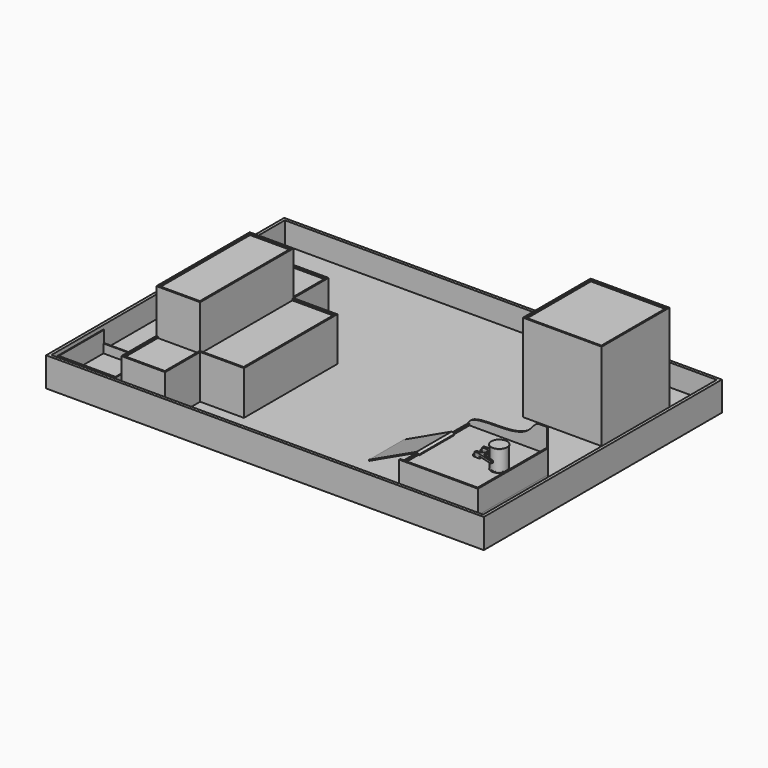
from build123d import *

# Parameters (mm, degrees)
F0_R      = 27.2
F1_DEPTH  = 2.83
F2_R      = 26.4
F3_DEPTH  = 67.36
F4_R      = 27.2
F5_DEPTH  = 2.83
F9_W      = 270
F9_H      = 300
F10_DEPTH = 72
F12_DEPTH = 15
F14_DEPTH = 5
F15_W     = 5
F15_H     = 290
F16_DEPTH = 5
F17_W     = 1500
F17_H     = 1020
F18_DEPTH = 25
F19_W     = 270
F19_H     = 290
F20_DEPTH = 300
F21_W     = 260
F21_H     = 280
F22_DEPTH = 5
F23_W     = 1500
F23_H     = 1020
F23_W_2   = 1480
F23_H_2   = 1000
F24_DEPTH = 75
F26_DEPTH = 150
F27_W     = 150
F27_H     = 400
F28_DEPTH = 150
F29_W     = 140
F29_H     = 390
F30_DEPTH = 5
F31_W     = 140
F31_H     = 145
F31_W_2   = 145
F31_H_2   = 390
F32_DEPTH = 5
F33_R     = 3
F34_DEPTH = 4
F35_R     = 3.99999
F35_2_R   = 3.99999
F36_R     = 3
F37_DEPTH = 8
F38_R     = 3
F39_DEPTH = 8
F40_R     = 3
F40_R_2   = 2.5
F41_DEPTH = 3
F42_R     = 3
F42_R_2   = 2.5
F43_DEPTH = 3
F45_DEPTH = 270.001
F46_W     = 200
F46_H     = 200
F46_W_2   = 194
F46_H_2   = 191
F47_DEPTH = 30
F49_DEPTH = 40
F52_DEPTH = 75
F50_R     = 2.5
F50_R_2   = 2.5911728926
F53_DEPTH = 7.25
F46_W_3   = 270
F46_H_3   = 300


# Not quite as in the source:
# - a fillet or chamfer is up to 0.001 mm smaller than in the source, because OpenCascade refuses the exact size
# - a feature names something its author has since deleted; it is built from what else it names


with BuildPart() as f1:
    # F0 (on Top) → F1 (new body)
    with BuildSketch(Plane.XY):
        Circle(F0_R)
    extrude(amount=F1_DEPTH)

    # F2 (on face) → F3 (join)
    with BuildSketch(Plane.XY.offset(2.83)):
        Circle(F2_R)
    extrude(amount=F3_DEPTH)

    # F4 (on face) → F5 (join)
    with BuildSketch(Plane.XY.offset(70.19)):
        Circle(F4_R)
    extrude(amount=F5_DEPTH)


with BuildPart() as f10:
    # F9 (on Top) → F10 (new body)
    with BuildSketch(Plane.XY):
        with Locations((-87.8, 0)):
            Rectangle(F9_W, F9_H)
    extrude(amount=-F10_DEPTH)

    # F11 (on face) → F12 (join)
    with BuildSketch(Plane.XY):
        Polygon((-222.8, -145), (-222.8, -150), (47.2, -150), (47.2, 150), (42.2, 150), (42.2, -145), align=None)
    extrude(amount=F12_DEPTH)

    # F13 (on face) → F14 (join)
    with BuildSketch(Plane(origin=(0, 150, 0), x_dir=(-1, 0, 0), z_dir=(0, 1, 0))):
        with BuildLine():
            Line((-21.3134280931, 81.3575685024), (-47.2, 81.3575685024))
            Line((-47.2, 81.3575685024), (-47.2, -72))
            Line((-47.2, -72), (222.8, -72))
            Line((222.8, -72), (222.8, 0))
            add(Edge.make_bspline(
                [(-21.3134280931, 81.3575685024), (-6.3059147253, 81.3822787863), (12.9585432644, 38.1268753575), (103.6097013063, 23.6068887567), (223.0224295336, 30.7718731823), (222.8, 0)],
                knots=[0, 0, 0, 0, 0.2487100673, 0.6151112321, 1, 1, 1, 1], degree=3))
        make_face()
    extrude(amount=-F14_DEPTH)

    # F15 (on face) → F16 (join)
    with BuildSketch(Plane.XY):
        with Locations((-220.3, 0)):
            Rectangle(F15_W, F15_H)
    extrude(amount=F16_DEPTH)

    # F17 (on face) → F18 (join)
    with BuildSketch(Plane(origin=(0, 0, -72), x_dir=(1, 0, 0), z_dir=(0, 0, -1))):
        with Locations((-602.8, -260)):
            Rectangle(F17_W, F17_H)
    extrude(amount=F18_DEPTH)

    # F19 (on face) → F20 (join)
    with BuildSketch(Plane.XY.offset(-72)):
        with Locations((-87.8, 525)):
            Rectangle(F19_W, F19_H)
    extrude(amount=F20_DEPTH)

    # F21 (on face) → F22 (cut)
    with BuildSketch(Plane.XY.offset(228)):
        with Locations((-87.8, 525)):
            Rectangle(F21_W, F21_H)
    extrude(amount=-F22_DEPTH, mode=Mode.SUBTRACT)

    # F23 (on face) → F24 (join)
    with BuildSketch(Plane.XY.offset(-72)):
        with Locations((-602.8, 260)):
            Rectangle(F23_W, F23_H)
        with Locations((-602.8, 260)):
            Rectangle(F23_W_2, F23_H_2, mode=Mode.SUBTRACT)
    extrude(amount=F24_DEPTH)

    # F25 (on face) → F26 (join)
    with BuildSketch(Plane.XY.offset(-72)):
        Polygon((-952.8, 460), (-1102.8, 460), (-1102.8, -240), (-952.8, -240), (-952.8, -90), (-802.8, -90), (-802.8, 310), (-952.8, 310), align=None)
    extrude(amount=F26_DEPTH)

    # F27 (on face) → F28 (join)
    with BuildSketch(Plane.XY.offset(78)):
        with Locations((-1027.8, 110)):
            Rectangle(F27_W, F27_H)
    extrude(amount=F28_DEPTH)

    # F29 (on face) → F30 (cut)
    with BuildSketch(Plane.XY.offset(228)):
        with Locations((-1027.8, 110)):
            Rectangle(F29_W, F29_H)
    extrude(amount=-F30_DEPTH, mode=Mode.SUBTRACT)

    # F31 (on face) → F32 (cut)
    with BuildSketch(Plane.XY.offset(78)):
        with Locations((-1027.8, 382.5)):
            Rectangle(F31_W, F31_H)
        with Locations((-880.3, 110)):
            Rectangle(F31_W_2, F31_H_2)
        with Locations((-1027.8, -162.5)):
            Rectangle(F31_W, F31_H)
    extrude(amount=-F32_DEPTH, mode=Mode.SUBTRACT)

    # F46 (on face) → F47 (join)
    with BuildSketch(Plane.XY.offset(-72)):
        with Locations((-1232.8, -130)):
            Rectangle(F46_W, F46_H)
        with Locations((-1232.8, -128.5)):
            Rectangle(F46_W_2, F46_H_2, mode=Mode.SUBTRACT)
    extrude(amount=F47_DEPTH)

    # F48 (on face) → F49 (join)
    with BuildSketch(Plane.XY.offset(-42)):
        Polygon((-1329.8, -30), (-1332.8, -30), (-1332.8, -230), (-1329.8, -230), (-1135.8, -230), (-1132.8, -230), (-1132.8, -30), (-1135.8, -30), (-1135.8, -224), (-1329.8, -224), align=None)
    extrude(amount=F49_DEPTH)


with BuildPart() as f34:
    # F33 (on offset) → F34 (new body, symmetric)
    with BuildSketch(Plane.XY.offset(25)):
        with BuildLine():
            Line((-55, -12), (-74.5, -12))
            Line((-74.5, -12), (-74.5, -13))
            Line((-74.5, -13), (-65.6457513111, -13))
            ThreePointArc((-65.6457513111, -13), (-67, -16), (-65.6457513111, -19))
            Line((-65.6457513111, -19), (-74.5, -19))
            Line((-74.5, -19), (-74.5, -20))
            Line((-74.5, -20), (-55, -20))
            ThreePointArc((-55, -20), (-51, -16), (-55, -12))
        make_face()
        with Locations((-63, -16)):
            Circle(F33_R, mode=Mode.SUBTRACT)
        with Locations((-55, -16)):
            Circle(F33_R, mode=Mode.SUBTRACT)
    extrude(amount=F34_DEPTH, both=True)

    # F35 (radius 4 in the source; OpenCascade refuses exactly that, so slightly less here)
    f35_edges = [f34.edges().sort_by_distance(p)[0] for p in [
        (-74.5, -19.5, 29),
        (-74.5, -12.5, 29),
        (-74.5, -19.5, 21),
        (-74.5, -12.5, 21),
    ]]
    fillet(f35_edges, radius=F35_R)

    # F36 (on face) → F37 (join, through all)
    with BuildSketch(Plane.XZ.offset(20)):
        with Locations((-70.5, 25)):
            Circle(F36_R)
    extrude(amount=-F37_DEPTH)

    # F42 (on offset) → F43 (join, symmetric)
    with BuildSketch(Plane.XY.offset(25)):
        with Locations((-63, -16)):
            Circle(F42_R)
        with Locations((-63, -16)):
            Circle(F42_R_2, mode=Mode.SUBTRACT)
        with Locations((-55, -16)):
            Circle(F42_R)
        with Locations((-55, -16)):
            Circle(F42_R_2, mode=Mode.SUBTRACT)
    extrude(amount=F43_DEPTH, both=True)


with BuildPart() as f34b:
    # F33 (on offset) → F34, piece 2 (new body, symmetric)
    with BuildSketch(Plane.XY.offset(25)):
        with BuildLine():
            Line((-74.5, 13), (-74.5, 12))
            Line((-74.5, 12), (-55, 12))
            ThreePointArc((-55, 12), (-51, 16), (-55, 20))
            Line((-55, 20), (-74.5, 20))
            Line((-74.5, 20), (-74.5, 19))
            Line((-74.5, 19), (-65.6457513111, 19))
            ThreePointArc((-65.6457513111, 19), (-67, 16), (-65.6457513111, 13))
            Line((-65.6457513111, 13), (-74.5, 13))
        make_face()
        with Locations((-63, 16)):
            Circle(F33_R, mode=Mode.SUBTRACT)
        with Locations((-55, 16)):
            Circle(F33_R, mode=Mode.SUBTRACT)
    extrude(amount=F34_DEPTH, both=True)

    # F35#2 (radius 4 in the source; OpenCascade refuses exactly that, so slightly less here)
    f35_2_edges = [f34b.edges().sort_by_distance(p)[0] for p in [
        (-74.5, 12.5, 29),
        (-74.5, 19.5, 29),
        (-74.5, 19.5, 21),
        (-74.5, 12.5, 21),
    ]]
    fillet(f35_2_edges, radius=F35_2_R)

    # F38 (on face) → F39 (join, through all)
    with BuildSketch(Plane(origin=(0, 20, 0), x_dir=(-1, 0, 0), z_dir=(0, 1, 0))):
        with Locations((70.5, 25)):
            Circle(F38_R)
    extrude(amount=-F39_DEPTH)

    # F40 (on offset) → F41 (join, symmetric)
    with BuildSketch(Plane.XY.offset(25)):
        with Locations((-55, 16)):
            Circle(F40_R)
        with Locations((-55, 16)):
            Circle(F40_R_2, mode=Mode.SUBTRACT)
        with Locations((-63, 16)):
            Circle(F40_R)
        with Locations((-63, 16)):
            Circle(F40_R_2, mode=Mode.SUBTRACT)
    extrude(amount=F41_DEPTH, both=True)


with BuildPart() as f45_tool:
    # F44 (on face) → F45 (new body, through all)
    with BuildSketch(Plane(origin=(0, 20, 0), x_dir=(-1, 0, 0), z_dir=(0, 1, 0))):
        with BuildLine():
            Line((71.5, 26), (71.5, 27.2912878475))
            ThreePointArc((71.5, 27.2912878475), (70.5, 27.5), (69.5, 27.2912878475))
            Line((69.5, 27.2912878475), (69.5, 26))
            Line((69.5, 26), (68.2087121525, 26))
            ThreePointArc((68.2087121525, 26), (68, 25), (68.2087121525, 24))
            Line((68.2087121525, 24), (69.5, 24))
            Line((69.5, 24), (69.5, 22.7087121525))
            ThreePointArc((69.5, 22.7087121525), (70.5, 22.5), (71.5, 22.7087121525))
            Line((71.5, 22.7087121525), (71.5, 24))
            Line((71.5, 24), (72.7912878475, 24))
            ThreePointArc((72.7912878475, 24), (73, 25), (72.7912878475, 26))
            Line((72.7912878475, 26), (71.5, 26))
        make_face()
    extrude(amount=-F45_DEPTH)


with BuildPart() as f34_1:
    add(f34.part)

    # F45: cut by f45_tool
    add(f45_tool.part, mode=Mode.SUBTRACT)


with BuildPart() as f34b_1:
    add(f34b.part)

    # F45: cut by f45_tool
    add(f45_tool.part, mode=Mode.SUBTRACT)


with BuildPart() as f52:
    # F51 (on Front) → F52 (new body, symmetric)
    with BuildSketch(Plane.XZ):
        Polygon((-386.7824421201, -69.2883481869), (-385.4991087867, -72), (-222.8, 5), (-222.8, 8.3190101902), align=None)
        Polygon((-222.8, 8.3190101902), (-222.8, 5), (-214.1397459622, 0), (-214.1397459622, 3.3190101902), align=None)
    extrude(amount=F52_DEPTH, both=True)


with BuildPart() as f53:
    # F50 (on face) → F53 (new body)
    with BuildSketch(Plane.XY.offset(29)):
        with BuildLine():
            Line((-57.4573915874, 20), (-68.4364587069, 20))
            Line((-68.4364587069, 20), (-68.4364587069, 12))
            Line((-68.4364587069, 12), (-49.8686146774, 12))
            Line((-49.8686146774, 12), (-36.8316546082, 0))
            Line((-36.8316546082, 0), (-49.8686146774, -12))
            Line((-49.8686146774, -12), (-68.4364587069, -12))
            Line((-68.4364587069, -12), (-68.4364587069, -20))
            Line((-68.4364587069, -20), (-57.4573915874, -20))
            Line((-57.4573915874, -20), (-0.6334627534, -35.2385337049))
            Line((-0.6334627534, -35.2385337049), (1.4669361943, -28.5544645366))
            Line((1.4669361943, -28.5544645366), (-38.1995291524, -17.9170661457))
            Line((-38.1995291524, -17.9170661457), (-26.8717848949, -4.2127397926))
            ThreePointArc((-26.8717848949, -4.2127397926), (-27.2, 0), (-26.8717848949, 4.2127397926))
            Line((-26.8717848949, 4.2127397926), (-38.1995291524, 17.9170661457))
            Line((-38.1995291524, 17.9170661457), (1.4669361943, 28.5544645366))
            Line((1.4669361943, 28.5544645366), (-0.6334627534, 35.2385337049))
            Line((-0.6334627534, 35.2385337049), (-57.4573915874, 20))
        make_face()
        with Locations((-63, -16)):
            Circle(F50_R, mode=Mode.SUBTRACT)
        with Locations((-55, -16)):
            Circle(F50_R, mode=Mode.SUBTRACT)
        with Locations((-3.8701845333, -30.5875726044)):
            Circle(F50_R, mode=Mode.SUBTRACT)
        with Locations((-31.9093577564, 0)):
            Circle(F50_R, mode=Mode.SUBTRACT)
        with Locations((-63, 16)):
            Circle(F50_R, mode=Mode.SUBTRACT)
        with Locations((-55, 16)):
            Circle(F50_R, mode=Mode.SUBTRACT)
        with Locations((-3.8701845333, 30.5875726044)):
            Circle(F50_R_2, mode=Mode.SUBTRACT)
    extrude(amount=F53_DEPTH)


with BuildPart() as f53b:
    # F46 (on face) → F53, piece 2 (new body)
    with BuildSketch(Plane.XY.offset(-72)):
        with Locations((-87.8, 0)):
            Rectangle(F46_W_3, F46_H_3)
    extrude(amount=F53_DEPTH)


solid = Compound([f1.part, f10.part, f34_1.part, f34b_1.part, f52.part, f53.part, f53b.part])
